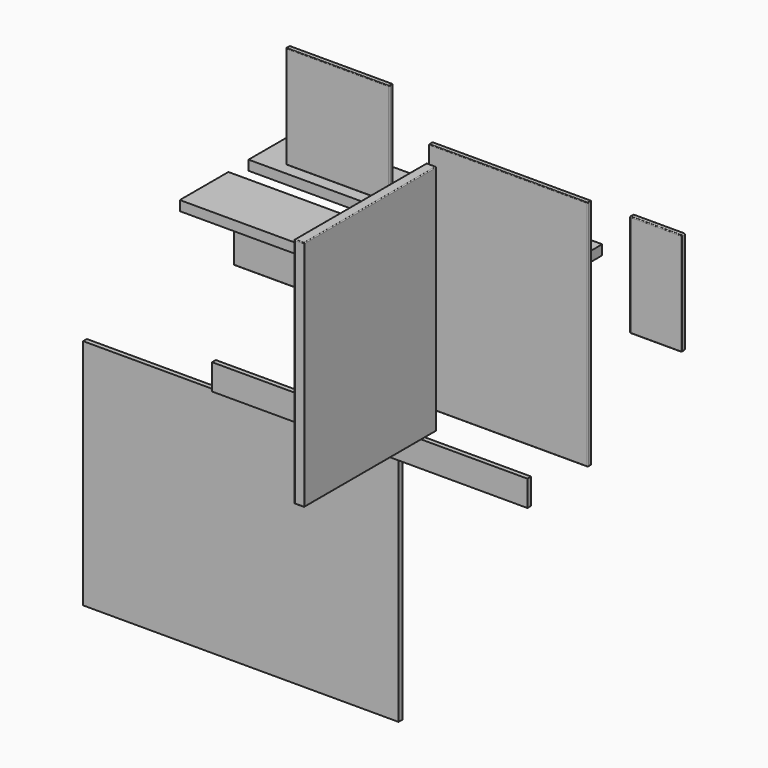
from build123d import *

# Parameters (mm, degrees)
F0_W         = 615
F0_H         = 900
F1_DEPTH     = 18
F2_R         = 2.5
F0_W_2       = 400
F0_H_2       = 398
F3_DEPTH     = 18
F0_W_3       = 600
F0_H_3       = 200
F4_R         = 2.5
F4_2_R       = 2.5
F5_W         = 1180
F5_H         = 235
F6_DEPTH     = 38
F5_W_2       = 595
F0_W_4       = 1220
F0_H_4       = 100
F7_DEPTH     = 18
F0_W_5       = 200
F8_DEPTH     = 18
F9_R         = 3
F10_W        = 1220
F10_H        = 900
F11_DEPTH    = 18
F12_W        = 640
F12_H        = 900
F13_DEPTH    = 38
F14_R        = 3
F15_R        = 3
F16_T1_DEPTH = 47
F17_T1_DEPTH = 47


# Not quite as in the source:
# - a fillet or chamfer that OpenCascade refuses, or shapes differently, is made with other operations: its cross-section is extruded or revolved along the edge and cut away or added


with BuildPart() as f1:
    # F0 (on Front) → F1 (new body)
    with BuildSketch(Plane.XZ):
        with Locations((-86.9357179105, -100.3156214945)):
            Rectangle(F0_W, F0_H)
    extrude(amount=F1_DEPTH)

    # F2
    f2_edges = [f1.edges().sort_by_distance(p)[0] for p in [
        (-86.935718, -18, 349.684379),
        (-394.435718, -18, -100.315621),
        (220.564282, -18, -100.315621),
        (-86.935718, -18, -550.315621),
        (220.564282, -9, 349.684379),
        (-394.435718, -9, 349.684379),
        (220.564282, -9, -550.315621),
        (-394.435718, -9, -550.315621),
        (-394.435718, 0, -100.315621),
        (-86.935718, 0, -550.315621),
        (-86.935718, 0, 349.684379),
        (220.564282, 0, -100.315621),
    ]]
    fillet(f2_edges, radius=F2_R)


with BuildPart() as f3:
    # F0 (on Front) → F3 (new body)
    with BuildSketch(Plane.XZ):
        with Locations((-747.0718502998, 298.6571630239)):
            Rectangle(F0_W_2, F0_H_2)
    extrude(amount=F3_DEPTH)

    # F4
    f4_edges = [f3.edges().sort_by_distance(p)[0] for p in [
        (-547.07185, -9, 497.657163),
        (-947.07185, -9, 497.657163),
        (-747.07185, 0, 497.657163),
        (-747.07185, -18, 497.657163),
        (-947.07185, -18, 298.657163),
        (-747.07185, -18, 99.657163),
        (-547.07185, -18, 298.657163),
        (-947.07185, -9, 99.657163),
        (-547.07185, -9, 99.657163),
        (-747.07185, 0, 99.657163),
        (-547.07185, 0, 298.657163),
        (-947.07185, 0, 298.657163),
    ]]
    fillet(f4_edges, radius=F4_R)


with BuildPart() as f3b:
    # F0 (on Front) → F3, piece 2 (new body)
    with BuildSketch(Plane.XZ):
        with Locations((-850.0371694565, -208.005541563)):
            Rectangle(F0_W_3, F0_H_3)
    extrude(amount=F3_DEPTH)

    # F4#2
    f4_2_edges = [f3b.edges().sort_by_distance(p)[0] for p in [
        (-550.037169, -9, -108.005542),
        (-1150.037169, -9, -108.005542),
        (-850.037169, 0, -108.005542),
        (-850.037169, -18, -108.005542),
        (-1150.037169, -18, -208.005542),
        (-850.037169, -18, -308.005542),
        (-550.037169, -18, -208.005542),
        (-1150.037169, -9, -308.005542),
        (-550.037169, -9, -308.005542),
        (-850.037169, 0, -308.005542),
        (-550.037169, 0, -208.005542),
        (-1150.037169, 0, -208.005542),
    ]]
    fillet(f4_2_edges, radius=F4_2_R)


with BuildPart() as f6:
    # F5 (on Top) → F6 (new body)
    with BuildSketch(Plane.XY):
        with Locations((-539.8566797376, 147.1251488424)):
            Rectangle(F5_W, F5_H)
    extrude(amount=F6_DEPTH)


with BuildPart() as f6b:
    # F5 (on Top) → F6, piece 2 (new body)
    with BuildSketch(Plane.XY):
        with Locations((-829.3576383591, -188.9490556717)):
            Rectangle(F5_W_2, F5_H)
    extrude(amount=F6_DEPTH)


with BuildPart() as f7:
    # F0 (on Front) → F7 (new body)
    with BuildSketch(Plane.XZ):
        with Locations((-622.8565120697, -715.9183740616)):
            Rectangle(F0_W_4, F0_H_4)
    extrude(amount=F7_DEPTH)


with BuildPart() as f8:
    # F0 (on Front) → F8 (new body)
    with BuildSketch(Plane.XZ):
        with Locations((483.1862807274, 157.4477581084)):
            Rectangle(F0_W_5, F0_H_2)
    extrude(amount=F8_DEPTH)

    # F9
    f9_edges = [f8.edges().sort_by_distance(p)[0] for p in [
        (483.186281, 0, 356.447758),
        (383.186281, 0, 157.447758),
        (483.186281, 0, -41.552242),
        (583.186281, 0, 157.447758),
        (483.186281, -18, 356.447758),
        (383.186281, -18, 157.447758),
        (483.186281, -18, -41.552242),
        (583.186281, -18, 157.447758),
        (583.186281, -9, 356.447758),
        (583.186281, -9, -41.552242),
        (383.186281, -9, -41.552242),
        (383.186281, -9, 356.447758),
    ]]
    fillet(f9_edges, radius=F9_R)


with BuildPart() as f11:
    # F10 (on face) → F11 (new body)
    with BuildSketch(Plane(origin=(0, 0, 0), x_dir=(-1, 0, 0), z_dir=(0, 1, 0))):
        with Locations((1135.9129697084, -1218.4509566795)):
            Rectangle(F10_W, F10_H)
    extrude(amount=F11_DEPTH)


with BuildPart() as f13:
    # F12 (on Right) → F13 (new body)
    with BuildSketch(Plane.YZ):
        with Locations((-841.4287376404, 167.809658368)):
            Rectangle(F12_W, F12_H)
    extrude(amount=F13_DEPTH)

    # F14
    f14_edges = [f13.edges().sort_by_distance(p)[0] for p in [
        (38, -841.428738, 617.809658),
        (38, -1161.428738, 167.809658),
        (38, -841.428738, -282.190342),
        (38, -521.428738, 167.809658),
    ]]
    fillet(f14_edges, radius=F14_R)

    # F15
    f15_edges = [f13.edges().sort_by_distance(p)[0] for p in [
        (0, -841.428738, 617.809658),
        (0, -1161.428738, 167.809658),
        (0, -841.428738, -282.190342),
        (0, -521.428738, 167.809658),
    ]]
    fillet(f15_edges, radius=F15_R)

    # F16: fillet of radius 3 on 4 edges, made by hand

    # F16_s2 → F16_t1 (cut)
    with BuildSketch(Plane.YZ.offset(-4.5)):
        with BuildLine():
            ThreePointArc((-1158.4287376404, 617.809658368), (-1160.5500579839, 616.9309787115), (-1161.4287376404, 614.809658368))
            Line((-1161.4287376404, 614.809658368), (-1161.4287376404, 617.809658368))
            Line((-1161.4287376404, 617.809658368), (-1158.4287376404, 617.809658368))
        make_face()
        with BuildLine():
            ThreePointArc((-1161.4287376404, -279.190341632), (-1160.5500579839, -281.3116619756), (-1158.4287376404, -282.190341632))
            Line((-1158.4287376404, -282.190341632), (-1161.4287376404, -282.190341632))
            Line((-1161.4287376404, -282.190341632), (-1161.4287376404, -279.190341632))
        make_face()
    extrude(amount=F16_T1_DEPTH, mode=Mode.SUBTRACT)

    # F17: fillet of radius 3 on 4 edges, made by hand

    # F17_s2 → F17_t1 (cut)
    with BuildSketch(Plane.YZ.offset(-4.5)):
        with BuildLine():
            ThreePointArc((-521.4287376404, -279.190341632), (-522.3074172968, -281.3116619756), (-524.4287376404, -282.190341632))
            Line((-524.4287376404, -282.190341632), (-521.4287376404, -282.190341632))
            Line((-521.4287376404, -282.190341632), (-521.4287376404, -279.190341632))
        make_face()
        with BuildLine():
            ThreePointArc((-524.4287376404, 617.809658368), (-522.3074172968, 616.9309787115), (-521.4287376404, 614.809658368))
            Line((-521.4287376404, 614.809658368), (-521.4287376404, 617.809658368))
            Line((-521.4287376404, 617.809658368), (-524.4287376404, 617.809658368))
        make_face()
    extrude(amount=F17_T1_DEPTH, mode=Mode.SUBTRACT)


solid = Compound([f1.part, f3.part, f3b.part, f6.part, f6b.part, f7.part, f8.part, f11.part, f13.part])
